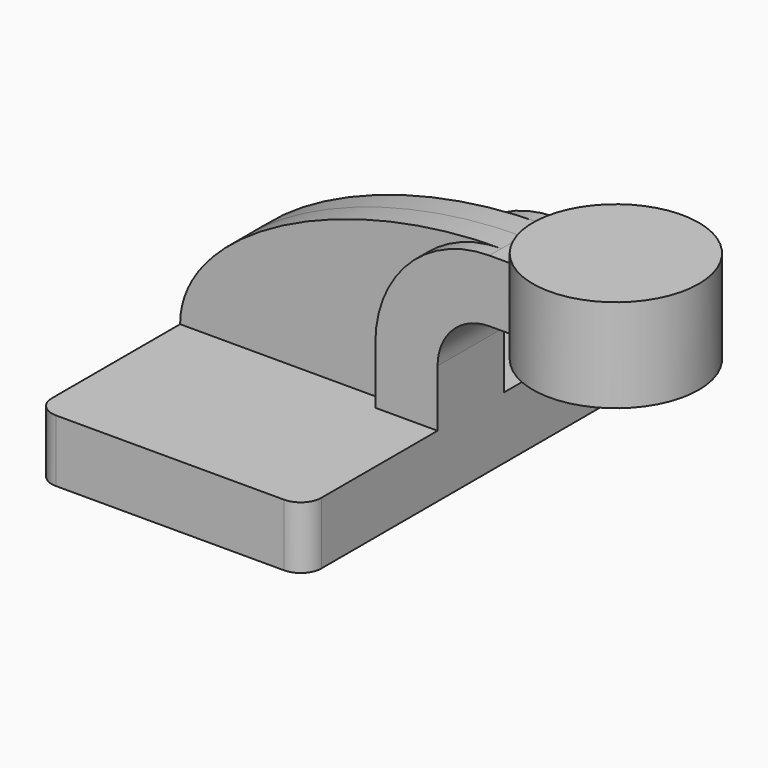
from build123d import *

# Parameters (mm, degrees)
F1_DEPTH = 63.5
F2_DEPTH = 12.7
F3_DEPTH = 8.0645
F5_R     = 6.35


# Not quite as in the source:
# - ends of sketch curves that miss each other by under 0.0002 mm in the source are joined


with BuildPart() as f1:
    # F0 (on Front) → F1 (new body, symmetric)
    with BuildSketch(Plane.XZ):
        Polygon((-41.275, -9.525), (41.275, -9.525), (41.275, 9.525), (22.225, 9.525), (-41.275, 9.525), align=None)
    extrude(amount=F1_DEPTH, both=True)

    # F0 (on Front) → F2 (join, symmetric)
    with BuildSketch(Plane.XZ):
        with BuildLine():
            Line((22.225, 9.525), (41.275, 9.525))
            Line((41.275, 9.525), (41.275, 27.0002))
            ThreePointArc((41.275, 27.0002), (45.9246798487, 38.2255201513), (57.15, 42.8752))
            Line((57.15, 42.8752), (60.325, 42.8752))
            Line((60.325, 42.8752), (60.325, 61.9252))
            Line((60.325, 61.9252), (57.15, 61.9252))
            ThreePointArc((57.15, 61.9252), (32.4542956671, 51.6959043329), (22.225, 27.0002))
            Line((22.225, 27.0002), (22.225, 9.525))
        make_face()
        Polygon((85.7250011283, 61.9252), (60.325, 61.9252), (60.325, 42.8752), (85.725, 42.8752), align=None)
    extrude(amount=F2_DEPTH, both=True)

    # F0 (on Front) → F3 (join, symmetric)
    with BuildSketch(Plane.XZ):
        with BuildLine():
            add(Edge.make_bspline(
                [(-41.275, 9.525), (-41.275, 36.3431351324), (6.7984250959, 61.9252), (57.15, 61.9252)],
                knots=[0, 0, 0, 0, 111.5045361635, 111.5045361635, 111.5045361635, 111.5045361635], degree=3))
            Line((-41.275, 9.525), (22.225, 9.525))
            Line((22.225, 9.525), (22.225, 27.0002))
            ThreePointArc((22.225, 27.0002), (32.4542956671, 51.6959043329), (57.15, 61.9252))
        make_face()
    extrude(amount=F3_DEPTH, both=True)

    # F0 (on Front) → F4 (revolve)
    with BuildSketch(Plane.XZ):
        Polygon((85.725, 66.675), (85.725, 61.9252), (85.725, 42.8752), (85.725, 38.1), (111.125, 38.1), (111.125, 66.675), align=None)
    revolve(axis=Axis((85.725, 0, 52.3875), (0, 0, 1)))

    # F5
    f5_edges = [f1.edges().sort_by_distance(p)[0] for p in [
        (41.275, -63.5, 0),
        (-41.275, -63.5, 0),
        (-41.275, 63.5, 0),
        (41.275, 63.5, 0),
    ]]
    fillet(f5_edges, radius=F5_R)


solid = f1.part
